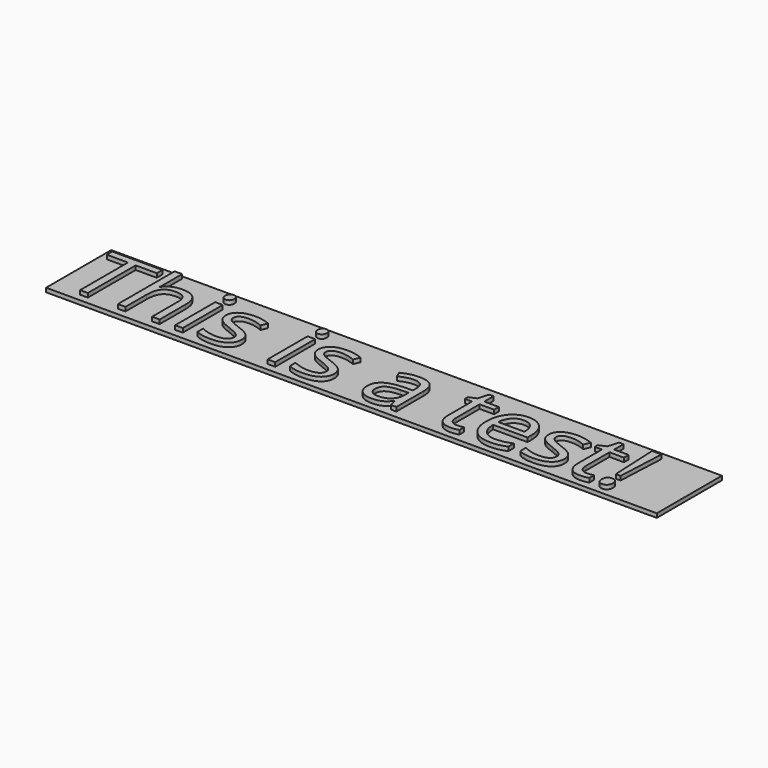
from build123d import *

# Parameters (mm, degrees)
F0_W         = 381
F0_H         = 50.8
F1_DEPTH     = 2.54
F2_TEXT_SIZE = 58.2521302729
F3_DEPTH     = 2.54


# Not quite as in the source:
# - Text() gives the source's letters only with a copy of the font that has no kerning and outlines rounded to 1/6400 em; it was checked with that copy


with BuildPart() as f1:
    # F0 (on Top) → F1 (new body)
    with BuildSketch(Plane.XY):
        with Locations((190.5, 25.4)):
            Rectangle(F0_W, F0_H)
    extrude(amount=F1_DEPTH)

    # F2 (on face) → F3 (join)
    with BuildSketch(Plane.XY.offset(2.54)):
        with Locations((3.9142849855, 4.5497911051)):
            Text('This is a test!', F2_TEXT_SIZE, font='Open Sans', text_align=(TextAlign.LEFT, TextAlign.BOTTOM))
    extrude(amount=F3_DEPTH)


solid = f1.part
